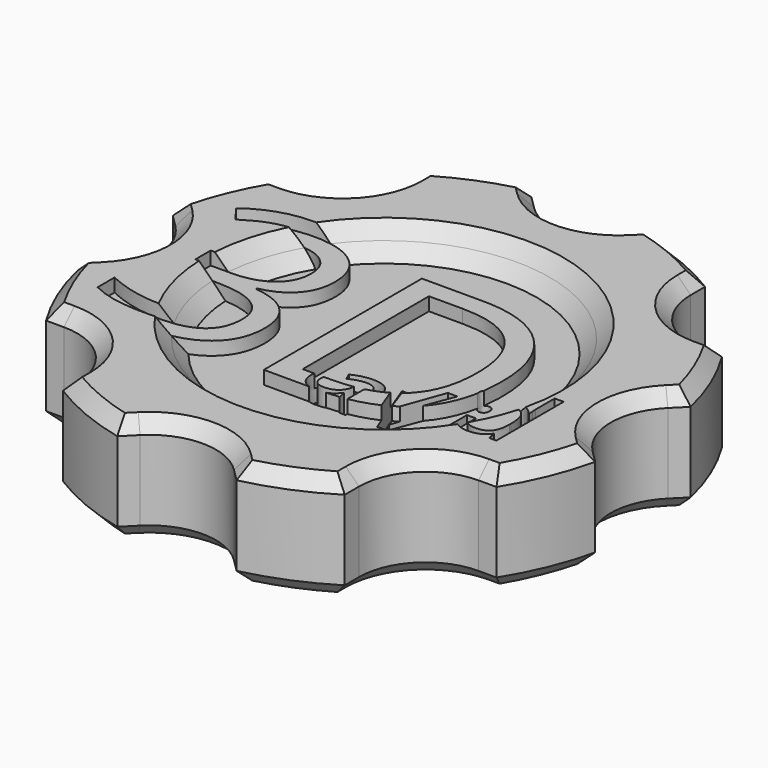
from build123d import *

# Parameters (mm, degrees)
F0_R         = 12.5
F1_DEPTH     = 8
F2_DEPTH     = 6
F3_SIZE      = 0.99999
F4_TEXT_SIZE = 20.8333333333
F5_DEPTH     = 1
F6_TEXT_SIZE = 8.3333333333
F7_DEPTH     = 3
F8_TEXT_SIZE = 20.8333333333
F9_DEPTH     = 1


# Not quite as in the source:
# - a fillet or chamfer is up to 0.001 mm smaller than in the source, because OpenCascade refuses the exact size
# - a feature names something its author has since deleted; it is built from what else it names
# - Text() gives the source's letters only with a copy of the font that has no kerning and outlines rounded to 1/6400 em; it was checked with that copy


with BuildPart() as f1:
    # F0 (on Top) → F1 (new body)
    with BuildSketch(Plane.XY):
        with BuildLine():
            Line((18.5355339059, 3.5355339059), (19.4895788083, 4.4895788083))
            ThreePointArc((19.4895788083, 4.4895788083), (18.4775906502, 7.6536686473), (16.9558249578, 10.6066017178))
            Line((16.9558249578, 10.6066017178), (15.6066017178, 10.6066017178))
            ThreePointArc((15.6066017178, 10.6066017178), (12.0710678119, 12.0710678119), (10.6066017178, 15.6066017178))
            Line((10.6066017178, 15.6066017178), (10.6066017178, 16.9558249578))
            ThreePointArc((10.6066017178, 16.9558249578), (7.6536686473, 18.4775906502), (4.4895788083, 19.4895788083))
            Line((4.4895788083, 19.4895788083), (3.5355339059, 18.5355339059))
            ThreePointArc((3.5355339059, 18.5355339059), (0, 17.0710678119), (-3.5355339059, 18.5355339059))
            Line((-3.5355339059, 18.5355339059), (-4.4895788083, 19.4895788083))
            ThreePointArc((-4.4895788083, 19.4895788083), (-7.6536686473, 18.4775906502), (-10.6066017178, 16.9558249578))
            Line((-10.6066017178, 16.9558249578), (-10.6066017178, 15.6066017178))
            ThreePointArc((-10.6066017178, 15.6066017178), (-12.0710678119, 12.0710678119), (-15.6066017178, 10.6066017178))
            Line((-15.6066017178, 10.6066017178), (-16.9558249578, 10.6066017178))
            ThreePointArc((-16.9558249578, 10.6066017178), (-18.4775906502, 7.6536686473), (-19.4895788083, 4.4895788083))
            Line((-19.4895788083, 4.4895788083), (-18.5355339059, 3.5355339059))
            ThreePointArc((-18.5355339059, 3.5355339059), (-17.0710678119, 0), (-18.5355339059, -3.5355339059))
            Line((-18.5355339059, -3.5355339059), (-19.4895788083, -4.4895788083))
            ThreePointArc((-19.4895788083, -4.4895788083), (-18.4775906502, -7.6536686473), (-16.9558249578, -10.6066017178))
            Line((-16.9558249578, -10.6066017178), (-15.6066017178, -10.6066017178))
            ThreePointArc((-15.6066017178, -10.6066017178), (-12.0710678119, -12.0710678119), (-10.6066017178, -15.6066017178))
            Line((-10.6066017178, -15.6066017178), (-10.6066017178, -16.9558249578))
            ThreePointArc((-10.6066017178, -16.9558249578), (-7.6536686473, -18.4775906502), (-4.4895788083, -19.4895788083))
            Line((-4.4895788083, -19.4895788083), (-3.5355339059, -18.5355339059))
            ThreePointArc((-3.5355339059, -18.5355339059), (0, -17.0710678119), (3.5355339059, -18.5355339059))
            Line((3.5355339059, -18.5355339059), (4.4895788083, -19.4895788083))
            ThreePointArc((4.4895788083, -19.4895788083), (7.6536686473, -18.4775906502), (10.6066017178, -16.9558249578))
            Line((10.6066017178, -16.9558249578), (10.6066017178, -15.6066017178))
            ThreePointArc((10.6066017178, -15.6066017178), (12.0710678119, -12.0710678119), (15.6066017178, -10.6066017178))
            Line((15.6066017178, -10.6066017178), (16.9558249578, -10.6066017178))
            ThreePointArc((16.9558249578, -10.6066017178), (18.4775906502, -7.6536686473), (19.4895788083, -4.4895788083))
            Line((19.4895788083, -4.4895788083), (18.5355339059, -3.5355339059))
            ThreePointArc((18.5355339059, -3.5355339059), (17.0710678119, 0), (18.5355339059, 3.5355339059))
        make_face()
        Circle(F0_R, mode=Mode.SUBTRACT)
    extrude(amount=F1_DEPTH)

    # F0 (on Top) → F2 (join)
    with BuildSketch(Plane.XY):
        Circle(F0_R)
    extrude(amount=F2_DEPTH)

    # F3 (size 1 in the source; OpenCascade refuses exactly that, so slightly less here)
    f3_edges = [f1.edges().sort_by_distance(p)[0] for p in [
        (-4.012556, -19.012556, 8),
        (0, -17.071068, 8),
        (4.012556, -19.012556, 8),
        (7.653669, -18.477591, 8),
        (10.606602, -16.281213, 8),
        (12.071068, -12.071068, 8),
        (16.281213, -10.606602, 8),
        (18.477591, -7.653669, 8),
        (19.012556, -4.012556, 8),
        (17.071068, 0, 8),
        (19.012556, 4.012556, 8),
        (18.477591, 7.653669, 8),
        (16.281213, 10.606602, 8),
        (12.071068, 12.071068, 8),
        (10.606602, 16.281213, 8),
        (7.653669, 18.477591, 8),
        (4.012556, 19.012556, 8),
        (0, 17.071068, 8),
        (-4.012556, 19.012556, 8),
        (-7.653669, 18.477591, 8),
        (-10.606602, 16.281213, 8),
        (-12.071068, 12.071068, 8),
        (-16.281213, 10.606602, 8),
        (-18.477591, 7.653669, 8),
        (-19.012556, 4.012556, 8),
        (-17.071068, 0, 8),
        (-19.012556, -4.012556, 8),
        (-18.477591, -7.653669, 8),
        (-16.281213, -10.606602, 8),
        (-12.071068, -12.071068, 8),
        (-10.606602, -16.281213, 8),
        (-7.653669, -18.477591, 8),
        (-12.5, 0, 8),
        (-4.012556, -19.012556, 0),
        (0, -17.071068, 0),
        (4.012556, -19.012556, 0),
        (7.653669, -18.477591, 0),
        (10.606602, -16.281213, 0),
        (12.071068, -12.071068, 0),
        (16.281213, -10.606602, 0),
        (18.477591, -7.653669, 0),
        (19.012556, -4.012556, 0),
        (17.071068, 0, 0),
        (19.012556, 4.012556, 0),
        (18.477591, 7.653669, 0),
        (16.281213, 10.606602, 0),
        (12.071068, 12.071068, 0),
        (10.606602, 16.281213, 0),
        (7.653669, 18.477591, 0),
        (4.012556, 19.012556, 0),
        (0, 17.071068, 0),
        (-4.012556, 19.012556, 0),
        (-7.653669, 18.477591, 0),
        (-10.606602, 16.281213, 0),
        (-12.071068, 12.071068, 0),
        (-16.281213, 10.606602, 0),
        (-18.477591, 7.653669, 0),
        (-19.012556, 4.012556, 0),
        (-17.071068, 0, 0),
        (-19.012556, -4.012556, 0),
        (-18.477591, -7.653669, 0),
        (-16.281213, -10.606602, 0),
        (-12.071068, -12.071068, 0),
        (-10.606602, -16.281213, 0),
        (-7.653669, -18.477591, 0),
        (-12.5, 0, 6),
    ]]
    chamfer(f3_edges, length=F3_SIZE)

    # F4 (on face) → F5 (join)
    with BuildSketch(Plane.XY.offset(6)):
        with Locations((-17, -7.5)):
            Text('3D', F4_TEXT_SIZE, font='Open Sans', text_align=(TextAlign.LEFT, TextAlign.BOTTOM))
    extrude(amount=F5_DEPTH)

    # F6 (on face) → F7 (cut, through all)
    with BuildSketch(Plane.XY.offset(8)):
        with Locations((-0.84765625, -7.5)):
            Text('avid', F6_TEXT_SIZE, font='Open Sans', text_align=(TextAlign.LEFT, TextAlign.BOTTOM))
    extrude(amount=-F7_DEPTH, mode=Mode.SUBTRACT)

    # F8 (on face) → F9 (cut, through all)
    with BuildSketch(Plane.XY.offset(8)):
        with Locations((-17, -7.5)):
            Text('3D', F8_TEXT_SIZE, font='Open Sans', text_align=(TextAlign.LEFT, TextAlign.BOTTOM))
    extrude(amount=-F9_DEPTH, mode=Mode.SUBTRACT)


solid = f1.part
